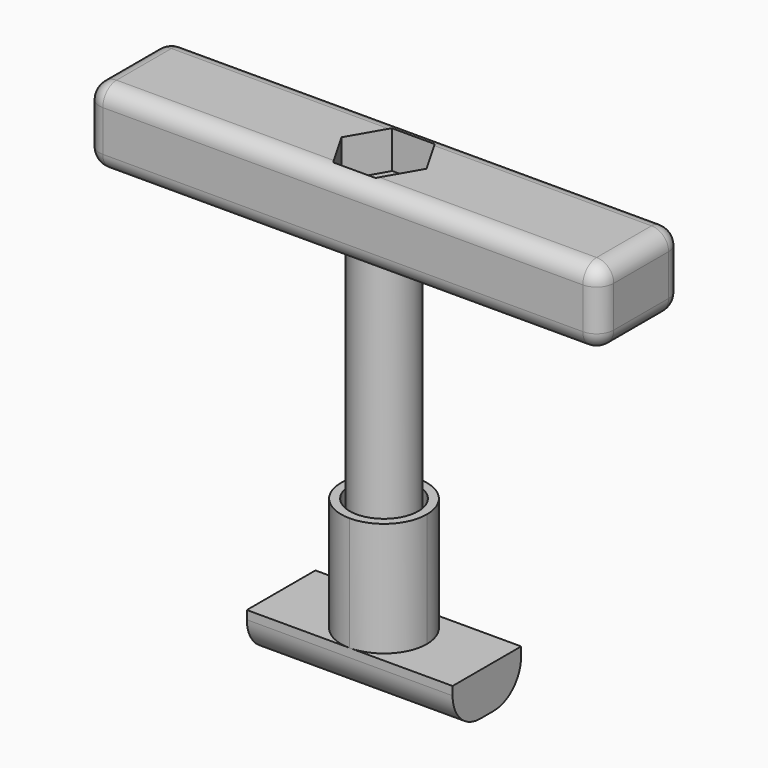
from build123d import *

# Parameters (mm, degrees)
F0_W         = 76.2
F0_H         = 15.24
F1_DEPTH     = 11.176
F4_DEPTH     = 5.588
F5_R         = 3.175
F6_DEPTH     = 11.176
F7_T1_DEPTH  = 6.096
F7_T3_DEPTH  = 10.16
F7_T5_DEPTH  = 71.12
F7_S9_W      = 2.54
F7_S9_H      = 2.54
F7_T10_DEPTH = 2.54
F7_S15_W     = 2.54
F7_S15_H     = 2.54
F7_T16_DEPTH = 2.54
F7_S21_W     = 2.54
F7_S21_H     = 2.54
F7_T22_DEPTH = 2.54
F7_S27_W     = 2.54
F7_S27_H     = 2.54
F7_T28_DEPTH = 2.54
F7_S33_W     = 2.54
F7_S33_H     = 2.54
F7_T34_DEPTH = 2.54
F7_S39_W     = 2.54
F7_S39_H     = 2.54
F7_T40_DEPTH = 2.54
F7_S45_W     = 2.54
F7_S45_H     = 2.54
F7_T46_DEPTH = 2.54
F7_S51_W     = 2.54
F7_S51_H     = 2.54
F7_T52_DEPTH = 2.54
F8_R         = 4.445
F9_DEPTH     = 50.8
F10_R        = 3.175
F11_DEPTH    = 61.976
F12_W        = 30.48
F12_H        = 12.7
F13_DEPTH    = 6.35
F14_R        = 5.08
F15_R        = 3.175
F16_DEPTH    = 71.6058239341
F17_W        = 9.715013206
F17_H        = 3.7662244022
F18_DEPTH    = 16.9285498559
F20_R        = 5.08
F21_DEPTH    = 16.9094242156
F22_R        = 3.81
F23_DEPTH    = 111.593618989


# Not quite as in the source:
# - a fillet or chamfer that OpenCascade refuses, or shapes differently, is made with other operations: its cross-section is extruded or revolved along the edge and cut away or added


with BuildPart() as f1:
    # F0 (on Top) → F1 (new body)
    with BuildSketch(Plane.XY):
        Rectangle(F0_W, F0_H)
    extrude(amount=F1_DEPTH)

    # F3 (on face) → F4 (cut)
    with BuildSketch(Plane.XY.offset(11.176)):
        Polygon((-3.15290982, -5.461), (3.15290982, -5.461), (6.3058196401, 0), (3.15290982, 5.461), (-3.15290982, 5.461), (-6.3058196401, 0), align=None)
    extrude(amount=-F4_DEPTH, mode=Mode.SUBTRACT)

    # F5 (on face) → F6 (cut)
    with BuildSketch(Plane.XY.offset(11.176)):
        Circle(F5_R)
    extrude(amount=-F6_DEPTH, mode=Mode.SUBTRACT)

    # F7: fillet of radius 2.54 on 12 edges, made by hand

    # F7_s2 → F7_t1 (cut)
    with BuildSketch(Plane.XY.offset(2.54)):
        with BuildLine():
            ThreePointArc((-35.56, -7.62), (-37.3560512242, -6.8760512242), (-38.1, -5.08))
            Line((-38.1, -5.08), (-38.1, -7.62))
            Line((-38.1, -7.62), (-35.56, -7.62))
        make_face()
        with BuildLine():
            ThreePointArc((-38.1, 5.08), (-37.3560512242, 6.8760512242), (-35.56, 7.62))
            Line((-35.56, 7.62), (-38.1, 7.62))
            Line((-38.1, 7.62), (-38.1, 5.08))
        make_face()
        with BuildLine():
            ThreePointArc((38.1, 5.08), (37.3560512242, 6.8760512242), (35.56, 7.62))
            Line((35.56, 7.62), (38.1, 7.62))
            Line((38.1, 7.62), (38.1, 5.08))
        make_face()
        with BuildLine():
            ThreePointArc((35.56, -7.62), (37.3560512242, -6.8760512242), (38.1, -5.08))
            Line((38.1, -5.08), (38.1, -7.62))
            Line((38.1, -7.62), (35.56, -7.62))
        make_face()
    extrude(amount=F7_T1_DEPTH, mode=Mode.SUBTRACT)

    # F7_s4 → F7_t3 (cut)
    with BuildSketch(Plane.XZ.offset(-5.08)):
        with BuildLine():
            ThreePointArc((38.1, 2.54), (37.3560512242, 0.7439487758), (35.56, 0))
            Line((35.56, 0), (38.1, 0))
            Line((38.1, 0), (38.1, 2.54))
        make_face()
        with BuildLine():
            ThreePointArc((-38.1, 8.636), (-37.3560512242, 10.4320512242), (-35.56, 11.176))
            Line((-35.56, 11.176), (-38.1, 11.176))
            Line((-38.1, 11.176), (-38.1, 8.636))
        make_face()
        with BuildLine():
            ThreePointArc((-38.1, 2.54), (-37.3560512242, 0.7439487758), (-35.56, 0))
            Line((-35.56, 0), (-38.1, 0))
            Line((-38.1, 0), (-38.1, 2.54))
        make_face()
        with BuildLine():
            ThreePointArc((38.1, 8.636), (37.3560512242, 10.4320512242), (35.56, 11.176))
            Line((35.56, 11.176), (38.1, 11.176))
            Line((38.1, 11.176), (38.1, 8.636))
        make_face()
    extrude(amount=F7_T3_DEPTH, mode=Mode.SUBTRACT)

    # F7_s6 → F7_t5 (cut)
    with BuildSketch(Plane.YZ.offset(-35.56)):
        with BuildLine():
            ThreePointArc((5.08, 11.176), (6.8760512242, 10.4320512242), (7.62, 8.636))
            Line((7.62, 8.636), (7.62, 11.176))
            Line((7.62, 11.176), (5.08, 11.176))
        make_face()
        with BuildLine():
            ThreePointArc((5.08, 0), (6.8760512242, 0.7439487758), (7.62, 2.54))
            Line((7.62, 2.54), (7.62, 0))
            Line((7.62, 0), (5.08, 0))
        make_face()
        with BuildLine():
            ThreePointArc((-7.62, 2.54), (-6.8760512242, 0.7439487758), (-5.08, 0))
            Line((-5.08, 0), (-7.62, 0))
            Line((-7.62, 0), (-7.62, 2.54))
        make_face()
        with BuildLine():
            ThreePointArc((-7.62, 8.636), (-6.8760512242, 10.4320512242), (-5.08, 11.176))
            Line((-5.08, 11.176), (-7.62, 11.176))
            Line((-7.62, 11.176), (-7.62, 8.636))
        make_face()
    extrude(amount=F7_T5_DEPTH, mode=Mode.SUBTRACT)


with BuildPart() as f7_tool8:
    # F7_s9 → F7_t10 (new body)
    with BuildSketch(Plane.XZ.offset(5.08)):
        with Locations((-36.83, 1.27)):
            Rectangle(F7_S9_W, F7_S9_H)
    extrude(amount=F7_T10_DEPTH)

    # F7_s11 → F7_t12 (revolve, cut)
    with BuildSketch(Plane(origin=(-35.56, -5.08, 2.54), x_dir=(0.7071067812, 0, 0.7071067812), z_dir=(0.7071067812, 0, -0.7071067812))):
        with BuildLine():
            ThreePointArc((0, -2.54), (2.54, 0), (0, 2.54))
            Line((0, 2.54), (0, -2.54))
        make_face()
    revolve(axis=Axis((-35.56, -5.08, 2.54), (0, -1, 0)), mode=Mode.SUBTRACT)


with BuildPart() as f1_1:
    add(f1.part)

    # F7_t7: cut F7_tool8
    add(f7_tool8.part, mode=Mode.SUBTRACT)


with BuildPart() as f7_tool14:
    # F7_s15 → F7_t16 (new body)
    with BuildSketch(Plane.XZ.offset(5.08)):
        with Locations((-36.83, 9.906)):
            Rectangle(F7_S15_W, F7_S15_H)
    extrude(amount=F7_T16_DEPTH)

    # F7_s17 → F7_t18 (revolve, cut)
    with BuildSketch(Plane(origin=(-35.56, -5.08, 8.636), x_dir=(0.7071067812, 0, -0.7071067812), z_dir=(-0.7071067812, 0, -0.7071067812))):
        with BuildLine():
            ThreePointArc((0, -2.54), (2.54, 0), (0, 2.54))
            Line((0, 2.54), (0, -2.54))
        make_face()
    revolve(axis=Axis((-35.56, -5.08, 8.636), (0, -1, 0)), mode=Mode.SUBTRACT)


with BuildPart() as f1_2:
    add(f1_1.part)

    # F7_t13: cut F7_tool14
    add(f7_tool14.part, mode=Mode.SUBTRACT)


with BuildPart() as f7_tool20:
    # F7_s21 → F7_t22 (new body)
    with BuildSketch(Plane.YZ.offset(-35.56)):
        with Locations((6.35, 1.27)):
            Rectangle(F7_S21_W, F7_S21_H)
    extrude(amount=-F7_T22_DEPTH)

    # F7_s23 → F7_t24 (revolve, cut)
    with BuildSketch(Plane(origin=(-35.56, 5.08, 2.54), x_dir=(0, -0.7071067812, 0.7071067812), z_dir=(0, -0.7071067812, -0.7071067812))):
        with BuildLine():
            ThreePointArc((0, -2.54), (2.54, 0), (0, 2.54))
            Line((0, 2.54), (0, -2.54))
        make_face()
    revolve(axis=Axis((-35.56, 5.08, 2.54), (-1, 0, 0)), mode=Mode.SUBTRACT)


with BuildPart() as f1_3:
    add(f1_2.part)

    # F7_t19: cut F7_tool20
    add(f7_tool20.part, mode=Mode.SUBTRACT)


with BuildPart() as f7_tool26:
    # F7_s27 → F7_t28 (new body)
    with BuildSketch(Plane.YZ.offset(-35.56)):
        with Locations((6.35, 9.906)):
            Rectangle(F7_S27_W, F7_S27_H)
    extrude(amount=-F7_T28_DEPTH)

    # F7_s29 → F7_t30 (revolve, cut)
    with BuildSketch(Plane(origin=(-35.56, 5.08, 8.636), x_dir=(0, -0.7071067812, -0.7071067812), z_dir=(0, 0.7071067812, -0.7071067812))):
        with BuildLine():
            ThreePointArc((0, -2.54), (2.54, 0), (0, 2.54))
            Line((0, 2.54), (0, -2.54))
        make_face()
    revolve(axis=Axis((-35.56, 5.08, 8.636), (-1, 0, 0)), mode=Mode.SUBTRACT)


with BuildPart() as f1_4:
    add(f1_3.part)

    # F7_t25: cut F7_tool26
    add(f7_tool26.part, mode=Mode.SUBTRACT)


with BuildPart() as f7_tool32:
    # F7_s33 → F7_t34 (new body)
    with BuildSketch(Plane.XZ.offset(5.08)):
        with Locations((36.83, 1.27)):
            Rectangle(F7_S33_W, F7_S33_H)
    extrude(amount=F7_T34_DEPTH)

    # F7_s35 → F7_t36 (revolve, cut)
    with BuildSketch(Plane(origin=(35.56, -5.08, 2.54), x_dir=(-0.7071067812, 0, 0.7071067812), z_dir=(0.7071067812, 0, 0.7071067812))):
        with BuildLine():
            ThreePointArc((0, -2.54), (2.54, 0), (0, 2.54))
            Line((0, 2.54), (0, -2.54))
        make_face()
    revolve(axis=Axis((35.56, -5.08, 2.54), (0, -1, 0)), mode=Mode.SUBTRACT)


with BuildPart() as f1_5:
    add(f1_4.part)

    # F7_t31: cut F7_tool32
    add(f7_tool32.part, mode=Mode.SUBTRACT)


with BuildPart() as f7_tool38:
    # F7_s39 → F7_t40 (new body)
    with BuildSketch(Plane.YZ.offset(35.56)):
        with Locations((6.35, 1.27)):
            Rectangle(F7_S39_W, F7_S39_H)
    extrude(amount=F7_T40_DEPTH)

    # F7_s41 → F7_t42 (revolve, cut)
    with BuildSketch(Plane(origin=(35.56, 5.08, 2.54), x_dir=(0, -0.7071067812, 0.7071067812), z_dir=(0, 0.7071067812, 0.7071067812))):
        with BuildLine():
            ThreePointArc((0, -2.54), (2.54, 0), (0, 2.54))
            Line((0, 2.54), (0, -2.54))
        make_face()
    revolve(axis=Axis((35.56, 5.08, 2.54), (1, 0, 0)), mode=Mode.SUBTRACT)


with BuildPart() as f1_6:
    add(f1_5.part)

    # F7_t37: cut F7_tool38
    add(f7_tool38.part, mode=Mode.SUBTRACT)


with BuildPart() as f7_tool44:
    # F7_s45 → F7_t46 (new body)
    with BuildSketch(Plane.YZ.offset(35.56)):
        with Locations((6.35, 9.906)):
            Rectangle(F7_S45_W, F7_S45_H)
    extrude(amount=F7_T46_DEPTH)

    # F7_s47 → F7_t48 (revolve, cut)
    with BuildSketch(Plane(origin=(35.56, 5.08, 8.636), x_dir=(0, -0.7071067812, -0.7071067812), z_dir=(0, -0.7071067812, 0.7071067812))):
        with BuildLine():
            ThreePointArc((0, -2.54), (2.54, 0), (0, 2.54))
            Line((0, 2.54), (0, -2.54))
        make_face()
    revolve(axis=Axis((35.56, 5.08, 8.636), (1, 0, 0)), mode=Mode.SUBTRACT)


with BuildPart() as f1_7:
    add(f1_6.part)

    # F7_t43: cut F7_tool44
    add(f7_tool44.part, mode=Mode.SUBTRACT)


with BuildPart() as f7_tool50:
    # F7_s51 → F7_t52 (new body)
    with BuildSketch(Plane.XZ.offset(5.08)):
        with Locations((36.83, 9.906)):
            Rectangle(F7_S51_W, F7_S51_H)
    extrude(amount=F7_T52_DEPTH)

    # F7_s53 → F7_t54 (revolve, cut)
    with BuildSketch(Plane(origin=(35.56, -5.08, 8.636), x_dir=(-0.7071067812, 0, -0.7071067812), z_dir=(-0.7071067812, 0, 0.7071067812))):
        with BuildLine():
            ThreePointArc((0, -2.54), (2.54, 0), (0, 2.54))
            Line((0, 2.54), (0, -2.54))
        make_face()
    revolve(axis=Axis((35.56, -5.08, 8.636), (0, -1, 0)), mode=Mode.SUBTRACT)


with BuildPart() as f1_8:
    add(f1_7.part)

    # F7_t49: cut F7_tool50
    add(f7_tool50.part, mode=Mode.SUBTRACT)

    # F8 (on face) → F9 (join)
    with BuildSketch(Plane(origin=(0, 0, 0), x_dir=(1, 0, 0), z_dir=(0, 0, -1))):
        Circle(F8_R)
    extrude(amount=F9_DEPTH)

    # F10 (on face) → F11 (cut)
    with BuildSketch(Plane.XY.offset(11.176)):
        Circle(F10_R)
    extrude(amount=-F11_DEPTH, mode=Mode.SUBTRACT)

    # F17 (on face) → F18 (cut)
    with BuildSketch(Plane(origin=(0, 6.35, 0), x_dir=(-1, 0, 0), z_dir=(0, 1, 0))):
        with Locations((0.1505874097, -48.9168877989)):
            Rectangle(F17_W, F17_H)
    extrude(amount=-F18_DEPTH, mode=Mode.SUBTRACT)

    # F22 (on face) → F23 (cut)
    with BuildSketch(Plane.XY.offset(11.176)):
        Circle(F22_R)
    extrude(amount=-F23_DEPTH, mode=Mode.SUBTRACT)


with BuildPart() as f13:
    # F12 (on face) → F13 (new body)
    with BuildSketch(Plane(origin=(0, 0, -50.8), x_dir=(1, 0, 0), z_dir=(0, 0, -1))):
        Rectangle(F12_W, F12_H)
    extrude(amount=F13_DEPTH)

    # F14
    f14_edges = [f13.edges().sort_by_distance(p)[0] for p in [
        (0, -6.35, -57.15),
        (0, 6.35, -57.15),
    ]]
    fillet(f14_edges, radius=F14_R)

    # F15 (on face) → F16 (cut)
    with BuildSketch(Plane.XY.offset(11.176)):
        Circle(F15_R)
    extrude(amount=-F16_DEPTH, mode=Mode.SUBTRACT)

    # F20 (on face) → F21 (join)
    with BuildSketch(Plane.XY.offset(-50.8)):
        with BuildLine():
            ThreePointArc((0, -6.35), (4.4901280605, -4.4901280605), (6.35, 0))
            ThreePointArc((6.35, 0), (4.4901280605, 4.4901280605), (0, 6.35))
            ThreePointArc((0, 6.35), (-6.35, 0), (0, -6.35))
        make_face()
        Circle(F20_R, mode=Mode.SUBTRACT)
    extrude(amount=F21_DEPTH)


solid = Compound([f1_8.part, f13.part])
